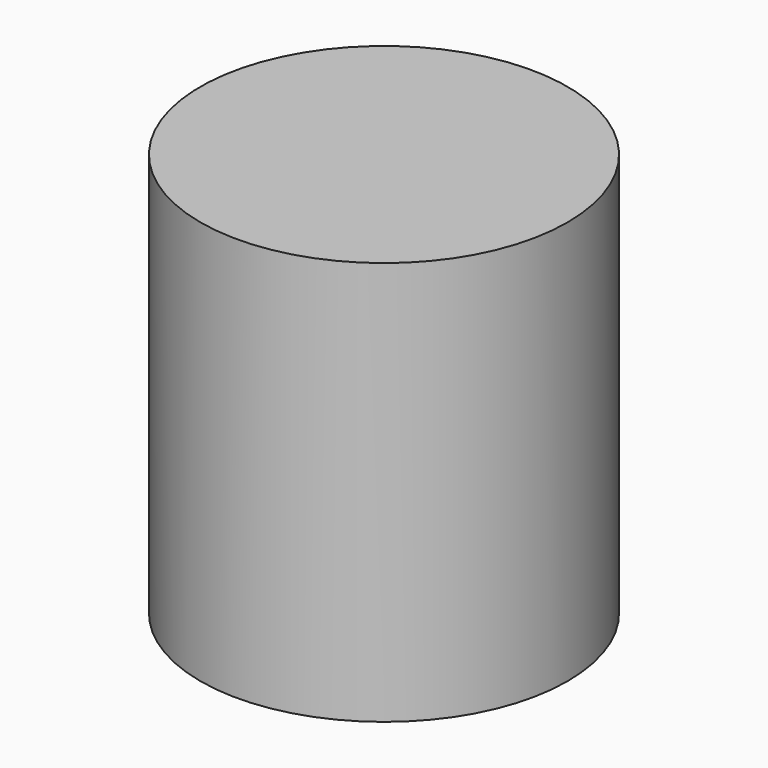
from build123d import *

# Parameters (mm, degrees)
F0_R     = 6.35
F1_DEPTH = 12.7
F3_R     = 6.35
F4_DEPTH = 1.27


# Not quite as in the source:
# - a feature names something its author has since deleted; it is built from what else it names


with BuildPart() as f1:
    # F0 (on Top) → F1 (new body)
    with BuildSketch(Plane.XY):
        Circle(F0_R)
        with BuildLine():
            ThreePointArc((-4.2518036763, -1.296221624), (0, 4.445), (4.2518036763, -1.296221624))
            Line((4.2518036763, -1.296221624), (-4.2518036763, -1.296221624))
        make_face(mode=Mode.SUBTRACT)
    extrude(amount=F1_DEPTH)

    # F3 (on offset) → F4 (join)
    with BuildSketch(Plane.XY.offset(12.7)):
        Circle(F3_R)
    extrude(amount=F4_DEPTH)


solid = f1.part
